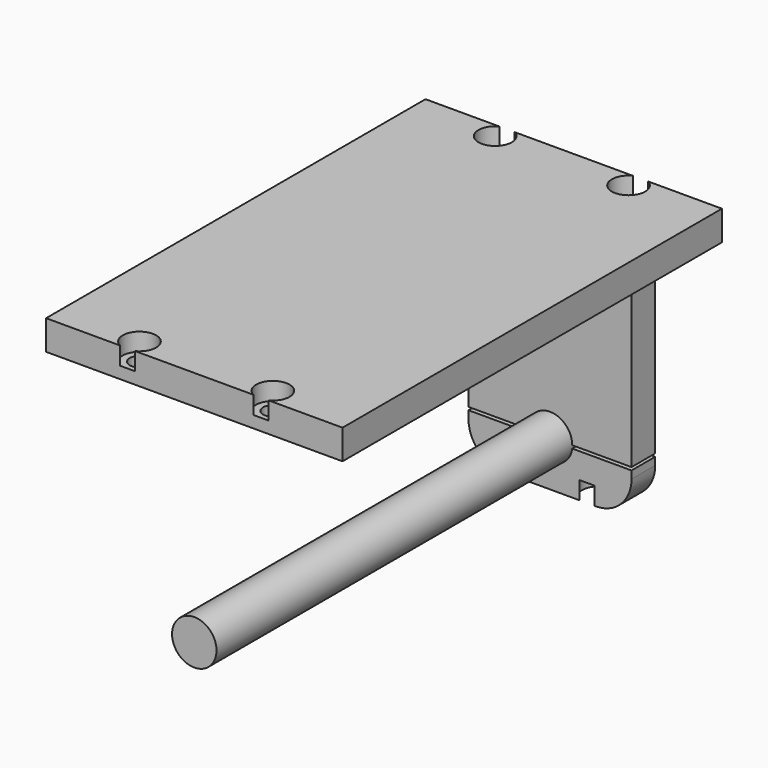
from build123d import *

# Parameters (mm, degrees)
F1_DEPTH        = 10
F3_D            = 5
F3_DEPTH        = 20
F3_TIP          = 1.5021515476
F4_W            = 55
F4_H            = 10
F4_R            = 2.5
F5_DEPTH        = 10
F7_D            = 6.6
F7_DEPTH        = 20
F7_CBORE_D      = 11.25
F7_CBORE_DEPTH  = 6
F7_TIP          = 1.9828400428
F10_D           = 5
F10_DEPTH       = 15
F10_TIP         = 1.5021515476
F12_D           = 6.6
F12_DEPTH       = 20
F12_CBORE_D     = 11.25
F12_CBORE_DEPTH = 6
F12_TIP         = 1.9828400428
F14_DEPTH       = 160


with BuildPart() as f1:
    # F0 (on Front) → F1 (new body)
    with BuildSketch(Plane.XZ):
        with BuildLine():
            Line((27.5, 70), (-27.5, 70))
            Line((-27.5, 70), (-27.5, 0))
            Line((-27.5, 0), (-7.5, 0))
            ThreePointArc((-7.5, 0), (0, 7.5), (7.5, 0))
            Line((7.5, 0), (27.5, 0))
            Line((27.5, 0), (27.5, 70))
        make_face()
    extrude(amount=F1_DEPTH)

    # F3
    with Locations(Plane.XY.offset(70)):
        with Locations((-22.5, -5), (22.5, -5)):
            Hole(F3_D / 2, depth=F3_DEPTH)
            with Locations((0, 0, -(F3_DEPTH + F3_TIP / 2))):  # 118° drill point
                Cone(0, F3_D / 2, F3_TIP, mode=Mode.SUBTRACT)

    # F10
    with Locations(Plane(origin=(0, 0, 0), x_dir=(1, 0, 0), z_dir=(0, 0, -1))):
        with Locations((-12.5, 5), (12.5, 5)):
            Hole(F10_D / 2, depth=F10_DEPTH)
            with Locations((0, 0, -(F10_DEPTH + F10_TIP / 2))):  # 118° drill point
                Cone(0, F10_D / 2, F10_TIP, mode=Mode.SUBTRACT)


with BuildPart() as f1b:
    # F0 (on Front) → F1, piece 2 (new body)
    with BuildSketch(Plane.XZ):
        with BuildLine():
            Line((27.5, -3.5663729752), (27.5, -1))
            Line((27.5, -1), (7.5, -1))
            ThreePointArc((7.5, -1), (0, -7.5663729752), (-7.5, -1))
            Line((-7.5, -1), (-27.5, -1))
            Line((-27.5, -1), (-27.5, -3.5663729752))
            ThreePointArc((-27.5, -3.5663729752), (-23.9852813742, -12.0516543494), (-15.5, -15.5663729752))
            Line((-15.5, -15.5663729752), (15.5, -15.5663729752))
            ThreePointArc((15.5, -15.5663729752), (23.9852813742, -12.0516543494), (27.5, -3.5663729752))
        make_face()
    extrude(amount=F1_DEPTH)

    # F12
    with Locations(Plane(origin=(0, 0, -15.5663729752), x_dir=(1, 0, 0), z_dir=(0, 0, -1))):
        with Locations((-12.5, 5), (12.5, 5)):
            CounterBoreHole(F12_D / 2, F12_CBORE_D / 2, F12_CBORE_DEPTH, depth=F12_DEPTH)
            with Locations((0, 0, -(F12_DEPTH + F12_TIP / 2))):  # 118° drill point
                Cone(0, F12_D / 2, F12_TIP, mode=Mode.SUBTRACT)


with BuildPart() as f5:
    # F4 (on face) → F5 (new body)
    with BuildSketch(Plane.XY.offset(70)):
        Polygon((-27.5, 0), (-50, 0), (-50, -80), (50, -80), (50, 0), (27.5, 0), (27.5, -10), (-27.5, -10), align=None)
        with Locations((0, -5)):
            Rectangle(F4_W, F4_H)
        with Locations((-22.5, -5)):
            Circle(F4_R, mode=Mode.SUBTRACT)
        with Locations((22.5, -5)):
            Circle(F4_R, mode=Mode.SUBTRACT)
    extrude(amount=F5_DEPTH)

    # F7
    with Locations(Plane.XY.offset(80)):
        with Locations((-22.5, -5), (22.5, -5)):
            CounterBoreHole(F7_D / 2, F7_CBORE_D / 2, F7_CBORE_DEPTH, depth=F7_DEPTH)
            with Locations((0, 0, -(F7_DEPTH + F7_TIP / 2))):  # 118° drill point
                Cone(0, F7_D / 2, F7_TIP, mode=Mode.SUBTRACT)

    # F8: F5 across face


with BuildPart() as f5_1:
    add(f5.part)
    add(f5.part.mirror(Plane(origin=(0, -80, 75), x_dir=(1, 0, 0), z_dir=(0, -1, 0))))


with BuildPart() as f14:
    # F13 (on face) → F14 (new body, through all)
    with BuildSketch(Plane(origin=(0, 0, 0), x_dir=(-1, 0, 0), z_dir=(0, 1, 0))):
        with BuildLine():
            ThreePointArc((-7.5, 0), (0, -7.5), (7.5, 0))
            ThreePointArc((7.5, 0), (0, 7.5), (-7.5, 0))
        make_face()
    extrude(amount=-F14_DEPTH)


solid = Compound([f1.part, f1b.part, f5_1.part, f14.part])
